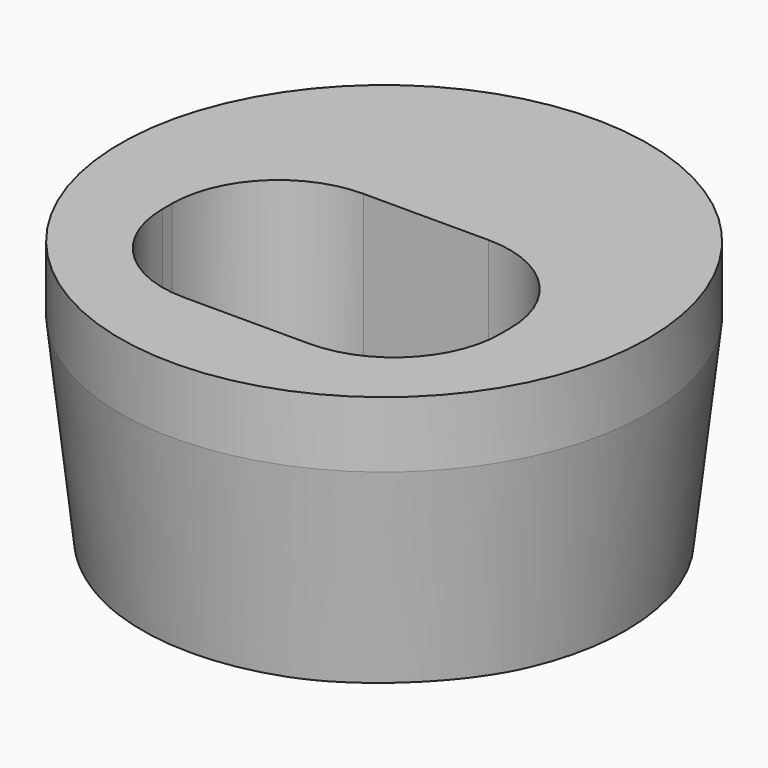
from build123d import *

# Parameters (mm, degrees)
F0_R         = 6
F1_DEPTH     = 6
F2_W         = 7.68
F2_H         = 5.1
F3_DEPTH     = 25
F4_R         = 2.4142135624
F5_SIZE2     = 0.5
F5_SIZE      = 4.5
F6_T1_DEPTH  = 2.8515728753
F6_T3_DEPTH  = 0.2715728753
F6_T6_ANGLE  = 90
F6_T8_ANGLE  = 90
F6_T10_ANGLE = 90
F6_T12_ANGLE = 90


# Not quite as in the source:
# - a fillet or chamfer that OpenCascade refuses, or shapes differently, is made with other operations: its cross-section is extruded or revolved along the edge and cut away or added


with BuildPart() as f1:
    # F0 (on Top) → F1 (new body)
    with BuildSketch(Plane.XY):
        Circle(F0_R)
    extrude(amount=F1_DEPTH)

    # F2 (on face) → F3 (cut)
    with BuildSketch(Plane.XY.offset(6)):
        with Locations((0, -1.3597839279)):
            Rectangle(F2_W, F2_H)
    extrude(amount=-F3_DEPTH, mode=Mode.SUBTRACT)

    # F4
    f4_edges = [f1.edges().sort_by_distance(p)[0] for p in [
        (-3.84, 1.190216, 3),
        (3.84, 1.190216, 3),
        (3.84, -3.909784, 3),
        (-3.84, -3.909784, 3),
    ]]
    fillet(f4_edges, radius=F4_R)

    # F5
    f5_edges = [f1.edges().sort_by_distance(p)[0] for p in [
        (-6, 0, 0),
    ]]
    f5_side = f1.faces().sort_by_distance((-6, 0, 3))[0]
    chamfer(f5_edges, length=F5_SIZE, length2=F5_SIZE2, reference=f5_side)

    # F6: fillet of radius 1.2795331881 on 8 edges, made by hand

    # F6_s2 → F6_t1 (cut)
    with BuildSketch(Plane.YZ.offset(-1.4257864376)):
        with BuildLine():
            ThreePointArc((-5.189317116, 0), (-4.2845505219, 0.374766594), (-3.9097839279, 1.2795331881))
            Line((-3.9097839279, 1.2795331881), (-3.9097839279, 0))
            Line((-3.9097839279, 0), (-5.189317116, 0))
        make_face()
        with BuildLine():
            ThreePointArc((2.4697492601, 0), (1.5649826661, 0.374766594), (1.1902160721, 1.2795331881))
            Line((1.1902160721, 1.2795331881), (1.1902160721, 0))
            Line((1.1902160721, 0), (2.4697492601, 0))
        make_face()
    extrude(amount=F6_T1_DEPTH, mode=Mode.SUBTRACT)

    # F6_s4 → F6_t3 (cut)
    with BuildSketch(Plane.XZ.offset(1.2239974903)):
        with BuildLine():
            ThreePointArc((-5.1195331881, 0), (-4.214766594, 0.374766594), (-3.84, 1.2795331881))
            Line((-3.84, 1.2795331881), (-3.84, 0))
            Line((-3.84, 0), (-5.1195331881, 0))
        make_face()
        with BuildLine():
            ThreePointArc((5.1195331881, 0), (4.214766594, 0.374766594), (3.84, 1.2795331881))
            Line((3.84, 1.2795331881), (3.84, 0))
            Line((3.84, 0), (5.1195331881, 0))
        make_face()
    extrude(amount=F6_T3_DEPTH, mode=Mode.SUBTRACT)

    # F6_s5 → F6_t6 (revolve, cut)
    with BuildSketch(Plane.YZ.offset(-1.4257864376)):
        with BuildLine():
            ThreePointArc((2.4697492601, 0), (1.5649826661, 0.374766594), (1.1902160721, 1.2795331881))
            Line((1.1902160721, 1.2795331881), (1.1902160721, 0))
            Line((1.1902160721, 0), (2.4697492601, 0))
        make_face()
    revolve(axis=Axis((-1.4257864376, -1.2239974903, 0), (0, 0, 1)), revolution_arc=F6_T6_ANGLE, mode=Mode.SUBTRACT)

    # F6_s7 → F6_t8 (revolve, cut)
    with BuildSketch(Plane.YZ.offset(-1.4257864376)):
        with BuildLine():
            ThreePointArc((-5.189317116, 0), (-4.2845505219, 0.374766594), (-3.9097839279, 1.2795331881))
            Line((-3.9097839279, 1.2795331881), (-3.9097839279, 0))
            Line((-3.9097839279, 0), (-5.189317116, 0))
        make_face()
    revolve(axis=Axis((-1.4257864376, -1.4955703655, 0), (0, 0, -1)), revolution_arc=F6_T8_ANGLE, mode=Mode.SUBTRACT)

    # F6_s9 → F6_t10 (revolve, cut)
    with BuildSketch(Plane.YZ.offset(1.4257864376)):
        with BuildLine():
            ThreePointArc((-5.189317116, 0), (-4.2845505219, 0.374766594), (-3.9097839279, 1.2795331881))
            Line((-3.9097839279, 1.2795331881), (-3.9097839279, 0))
            Line((-3.9097839279, 0), (-5.189317116, 0))
        make_face()
    revolve(axis=Axis((1.4257864376, -1.4955703655, 0), (0, 0, 1)), revolution_arc=F6_T10_ANGLE, mode=Mode.SUBTRACT)

    # F6_s11 → F6_t12 (revolve, cut)
    with BuildSketch(Plane.XZ.offset(1.2239974903)):
        with BuildLine():
            ThreePointArc((5.1195331881, 0), (4.214766594, 0.374766594), (3.84, 1.2795331881))
            Line((3.84, 1.2795331881), (3.84, 0))
            Line((3.84, 0), (5.1195331881, 0))
        make_face()
    revolve(axis=Axis((1.4257864376, -1.2239974903, 0), (0, 0, 1)), revolution_arc=F6_T12_ANGLE, mode=Mode.SUBTRACT)


solid = f1.part
